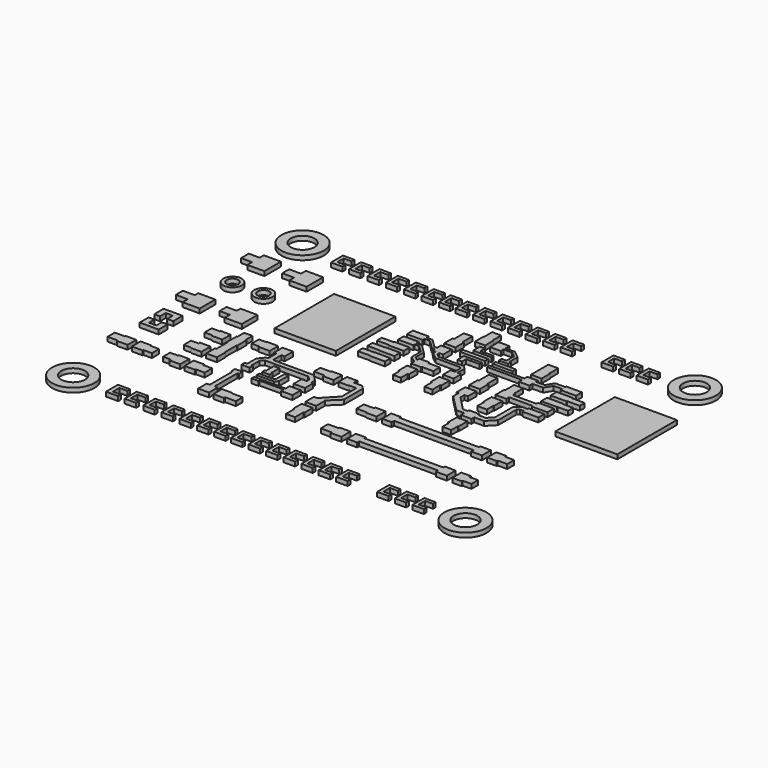
from build123d import *

# Parameters (mm, degrees)
F0_W     = 8.8383136317
F0_H     = 10.7280849479
F2_DEPTH = 0.635
F0_W_2   = 8.9478660375
F0_H_2   = 10.732548777
F0_W_3   = 3.4179408103
F0_H_3   = 0.6752701011
F0_W_4   = 1.5755221248
F0_H_4   = 1.3810726814
F0_W_5   = 1.7077755183
F0_H_5   = 1.243758481
F0_W_6   = 1.7230845988
F0_H_6   = 1.2770355679
F0_R     = 0.3036526341
F0_W_7   = 1.472780481
F0_H_7   = 1.2533185072
F0_R_2   = 0.3044951646
F0_W_8   = 1.8562953919
F0_H_8   = 0.8942730201
F0_W_9   = 1.5506837517
F0_H_9   = 0.9251098963
F0_W_10  = 1.4100596309
F0_H_10  = 0.5669312086
F0_W_11  = 1.561771147
F0_H_11  = 1.2164656073
F0_W_12  = 1.305432932
F0_H_12  = 1.5174094588
F0_W_13  = 1.1086538434
F0_H_13  = 1.3054329902
F0_W_14  = 1.5646023676
F0_H_14  = 1.2951530516
F0_W_15  = 1.2573283166
F0_H_15  = 1.1950880289
F0_W_16  = 1.378653571
F0_H_16  = 1.2574242428
F0_W_17  = 1.2773927301
F0_H_17  = 1.2361174449
F0_W_18  = 1.151248347
F0_H_18  = 1.3980204239
F0_W_19  = 3.6632483825
F0_H_19  = 0.4471028224
F0_W_20  = 1.1279918253
F0_H_20  = 1.2643169612
F0_W_21  = 1.2620901689
F0_H_21  = 2.1310206503
F0_W_22  = 1.202643849
F0_H_22  = 1.2692697346
F0_W_23  = 1.1741518974
F0_H_23  = 1.2878933921
F0_W_24  = 1.2717936188
F0_H_24  = 1.3373773545
F0_W_25  = 1.4900562819
F0_H_25  = 1.1629359797
F0_W_26  = 1.1306900997
F0_H_26  = 1.1970004998
F0_W_27  = 1.3690730557
F0_H_27  = 1.217473764
F0_W_28  = 1.0838713497
F0_H_28  = 1.3157110661
F0_W_29  = 1.3664499857
F0_H_29  = 0.4357985454
F0_W_30  = 1.2792297639
F0_H_30  = 0.5960047711
F1_R     = 3.0492368832
F1_R_2   = 1.7145
F3_DEPTH = 0.635
F1_R_3   = 1.3313448852
F1_R_4   = 0.8262831424
F1_R_5   = 1.3281430865
F1_R_6   = 0.8239920233
F1_R_7   = 3.048384159
F1_R_8   = 3.0501055082
F1_R_9   = 3.0482052647
F1_R_10  = 1.7111635464


# Not quite as in the source:
# - ends of sketch curves that miss each other by under 0.0002 mm in the source are joined
# - a feature names something its author has since deleted; it is built from what else it names


with BuildPart() as f2:
    # F0 (on Top) → F2 (new body)
    with BuildSketch(Plane.XY):
        with Locations((-10.1480917074, -1.0168242734)):
            Rectangle(F0_W, F0_H)
    extrude(amount=F2_DEPTH)


with BuildPart() as f2b:
    # F0 (on Top) → F2, piece 2 (new body)
    with BuildSketch(Plane.XY):
        with Locations((30.3083872423, -0.916500343)):
            Rectangle(F0_W_2, F0_H_2)
    extrude(amount=F2_DEPTH)


with BuildPart() as f2c:
    # F0 (on Top) → F2, piece 3 (new body)
    with BuildSketch(Plane.XY):
        with Locations((18.2702904567, -2.6805658126)):
            Rectangle(F0_W_3, F0_H_3)
        Polygon((15.1307059766, -0.3272882414), (15.1360724121, -1.9821051974), (16.4415054023, -1.9821051974), (16.4415054023, -0.3272882414), align=None)
        Polygon((19.9792608619, -2.3429307621), (19.9792608619, -3.0182008632), (19.9792608619, -3.1918291934), (22.220082581, -3.1918291934), (22.220082581, -2.0200230647), (19.9792608619, -2.0200230647), align=None)
        Polygon((15.1360724121, -1.9821051974), (15.0048257783, -1.9821051974), (15.0048257783, -3.5278119612), (16.5613200516, -3.5278119612), (16.5613200516, -3.0182008632), (16.5613200516, -2.3429307621), (16.5613200516, -1.9821051974), (16.4415054023, -1.9821051974), align=None)
    extrude(amount=F2_DEPTH)


with BuildPart() as f2d:
    # F0 (on Top) → F2, piece 4 (new body)
    with BuildSketch(Plane.XY):
        Polygon((-24.1649243981, 6.7577632144), (-26.6341436654, 6.7577632144), (-26.6341436654, 6.0122814029), (-26.6341436654, 4.6312087215), (-26.6341436654, 3.7751416676), (-24.1649243981, 3.7751416676), align=None)
        with Locations((-27.4219047278, 5.3217450622)):
            Rectangle(F0_W_4, F0_H_4)
    extrude(amount=F2_DEPTH)


with BuildPart() as f2e:
    # F0 (on Top) → F2, piece 5 (new body)
    with BuildSketch(Plane.XY):
        Polygon((-18.0774424225, 6.7577632144), (-20.5711107701, 6.7577632144), (-20.5711107701, 5.8749672025), (-20.5711107701, 4.6312087215), (-20.5711107701, 3.7751416676), (-18.0774424225, 3.7751416676), align=None)
        with Locations((-21.4249985293, 5.253087962)):
            Rectangle(F0_W_5, F0_H_5)
    extrude(amount=F2_DEPTH)


with BuildPart() as f2f:
    # F0 (on Top) → F2, piece 6 (new body)
    with BuildSketch(Plane.XY):
        Polygon((-24.1649243981, -5.0749327056), (-26.6341455281, -5.0749327056), (-26.6341455281, -5.6854607537), (-26.6341455281, -6.9624963216), (-26.6341455281, -7.8864200041), (-24.1649243981, -7.8864200041), align=None)
        with Locations((-27.4956878275, -6.3239785377)):
            Rectangle(F0_W_6, F0_H_6)
        with Locations((-27.8962515295, -6.3951537013)):
            Circle(F0_R, mode=Mode.SUBTRACT)
        with Locations((-27.8962515295, -6.3951537013)):
            Circle(F0_R)
    extrude(amount=F2_DEPTH)


with BuildPart() as f2g:
    # F0 (on Top) → F2, piece 7 (new body)
    with BuildSketch(Plane.XY):
        Polygon((-18.1018915027, -5.0504850224), (-20.5711107701, -5.0504850224), (-20.5711107701, -5.7091778144), (-20.5711107701, -6.9624963216), (-20.5711107701, -7.8864200041), (-18.1018915027, -7.8864200041), align=None)
        with Locations((-21.3075010106, -6.335837068)):
            Rectangle(F0_W_7, F0_H_7)
        with Locations((-21.5573497117, -6.3951537013)):
            Circle(F0_R_2, mode=Mode.SUBTRACT)
        with Locations((-21.5573497117, -6.3951537013)):
            Circle(F0_R_2)
    extrude(amount=F2_DEPTH)


with BuildPart() as f2h:
    # F0 (on Top) → F2, piece 8 (new body)
    with BuildSketch(Plane.XY):
        Polygon((19.9587028474, -3.7468951195), (19.9587028474, -3.9533996023), (19.9587028474, -4.5840349048), (19.9587028474, -4.8159109429), (22.220082581, -4.8159109429), (22.220082581, -3.7468951195), align=None)
        Polygon((15.0194698945, -9.1961659491), (15.0194698945, -8.5539119318), (14.3346317847, -8.5539119318), (12.3020727187, -6.4541599101), (12.3020727187, -5.7373908348), (11.4847198129, -5.7373908348), (11.4847198129, -6.742843182), (13.8865737244, -9.1961659491), align=None)
        Polygon((17.6625381124, -8.5858944803), (16.5613200516, -8.5858944803), (16.5613200516, -9.3020955101), (17.9853862302, -9.3020955101), (19.0944410861, -8.1543523612), (19.0944410861, -4.8597618444), (19.3846803159, -4.5840349048), (19.9587028474, -4.5840349048), (19.9587028474, -3.9533996023), (19.1347077489, -3.9533996023), (18.3828920126, -4.6720469973), (18.3828920126, -7.8655403551), align=None)
        Polygon((11.4847198129, -5.7373908348), (12.3020727187, -5.7373908348), (12.7952471375, -5.7373908348), (12.7952471375, -4.1965004057), (11.1816739663, -4.1965004057), (11.1816739663, -5.7373908348), align=None)
        Polygon((16.5613200516, -8.3131287247), (15.0194698945, -8.3131287247), (15.0194698945, -8.5539119318), (15.0194698945, -9.1961659491), (15.0194698945, -9.7933048382), (16.5613200516, -9.7933048382), (16.5613200516, -9.3020955101), (16.5613200516, -8.5858944803), align=None)
    extrude(amount=F2_DEPTH)


with BuildPart() as f2i:
    # F0 (on Top) → F2, piece 9 (new body)
    with BuildSketch(Plane.XY):
        Polygon((0.2071742638, 1.1828735005), (-1.987867523, 1.1828735005), (-1.987867523, 0.1507677225), (0.2071742638, 0.1507677225), (0.2071742638, 0.3949551319), (0.8484240971, 0.3949551319), (1.8542347467, -0.5398768699), (1.8542347467, -2.200213147), (2.7769438457, -2.8982465155), (2.7769438457, -3.4828390926), (4.2571197264, -3.4828390926), (4.2571197264, -3.3824450802), (5.9211971238, -3.3824450802), (5.9211971238, -2.2117714398), (4.2571197264, -2.2117714398), (4.2571197264, -1.9821051974), (2.7769438457, -1.9821051974), (2.7769438457, -2.3882756941), (2.2400394082, -1.9821051974), (2.2400394082, -0.4953329917), (0.995364855, 0.7406980731), (0.2071742638, 0.7406980731), align=None)
    extrude(amount=F2_DEPTH)


with BuildPart() as f2j:
    # F0 (on Top) → F2, piece 10 (new body)
    with BuildSketch(Plane.XY):
        with Locations((23.1571951881, 0.7704721793)):
            Rectangle(F0_W_8, F0_H_8)
        Polygon((22.2290474921, 1.3358424185), (19.9309624732, 1.3358424185), (19.9309624732, 0.2356950572), (22.2290474921, 0.2356950572), (22.2290474921, 0.3233356692), (22.2290474921, 1.2176086893), align=None)
    extrude(amount=F2_DEPTH)


with BuildPart() as f2k:
    # F0 (on Top) → F2, piece 11 (new body)
    with BuildSketch(Plane.XY):
        Polygon((0.2217109577, 2.9127409216), (-2.0460144151, 2.9127409216), (-2.0460144151, 1.8079516012), (0.2217109577, 1.8079516012), (0.2217109577, 2.1451261241), (0.2217109577, 2.5225197896), align=None)
        Polygon((3.6875456572, 0.4741872835), (3.1932978891, 0.4741872835), (3.1932978891, 0), (4.1236467659, -0.7333545946), (7.6851383783, -0.7333545946), (7.9177254811, -1.0095519247), (7.9177254811, -1.9821051974), (8.310216479, -1.9821051974), (8.310216479, -0.7042811485), (7.8159682453, -0.2681801561), (4.1963304393, -0.2681801561), (3.6875456572, 0.1533842151), align=None)
        Polygon((8.310216479, -1.9821051974), (7.9177254811, -1.9821051974), (7.3003736325, -1.9821051974), (7.3003736325, -3.3824450802), (8.8267270476, -3.3824450802), (8.8267270476, -1.9821051974), align=None)
        Polygon((2.6861303486, 2.047317801), (2.6861303486, 1.3202173682), (2.6861303486, 0.9452876402), (2.6861303486, 0.4741872835), (3.1932978891, 0.4741872835), (3.6875456572, 0.4741872835), (4.2571197264, 0.4741872835), (4.2571197264, 2.047317801), align=None)
        Polygon((1.0968204588, 2.5225197896), (0.2217109577, 2.5225197896), (0.2217109577, 2.1451261241), (1.0318105284, 2.1451261241), (2.2400394082, 0.9452876402), (2.6861303486, 0.9452876402), (2.6861303486, 1.3202173682), (2.3075305063, 1.3202173682), align=None)
    extrude(amount=F2_DEPTH)


with BuildPart() as f2l:
    # F0 (on Top) → F2, piece 12 (new body)
    with BuildSketch(Plane.XY):
        Polygon((11.3475334477, -0.1729048687), (11.3534005359, -1.9821051974), (12.6030265707, -1.9821051974), (12.5971594825, -0.1729048687), align=None)
        Polygon((11.3534005359, -1.9821051974), (11.1962100491, -1.9821051974), (11.1962100491, -3.5278121941), (12.7516370267, -3.5278121941), (12.7516370267, -1.9821051974), (12.6030265707, -1.9821051974), align=None)
    extrude(amount=F2_DEPTH)


with BuildPart() as f2m:
    # F0 (on Top) → F2, piece 13 (new body)
    with BuildSketch(Plane.XY):
        Polygon((0.1926377008, -3.9195087738), (-1.9442574121, -3.9195087738), (-1.9442574121, -3.9598466904), (-1.9442574121, -4.8703011125), (-1.9442574121, -4.9370778725), (0.1926377008, -4.9370778725), align=None)
        Polygon((-1.9442574121, -4.8703011125), (-1.9442574121, -3.9598466904), (-3.7691615199, -3.9657647046), (-3.766209022, -4.876209552), align=None)
    extrude(amount=F2_DEPTH)


with BuildPart() as f2n:
    # F0 (on Top) → F2, piece 14 (new body)
    with BuildSketch(Plane.XY):
        with Locations((23.0427468196, -1.0026553937)):
            Rectangle(F0_W_9, F0_H_9)
        Polygon((22.2674049437, -0.4488411068), (19.979858771, -0.4488411068), (19.979858771, -1.505690976), (22.2674049437, -1.505690976), (22.2674049437, -1.4652103418), (22.2674049437, -0.5401004455), align=None)
    extrude(amount=F2_DEPTH)


with BuildPart() as f2o:
    # F0 (on Top) → F2, piece 15 (new body)
    with BuildSketch(Plane.XY):
        Polygon((12.9254506901, 2.7643614449), (11.4117721096, 2.7643614449), (11.4117721096, 2.1974302363), (12.9254506901, 2.182893455), align=None)
        with Locations((10.7067422941, 2.4808958406)):
            Rectangle(F0_W_10, F0_H_10)
    extrude(amount=F2_DEPTH)


with BuildPart() as f2p:
    # F0 (on Top) → F2, piece 16 (new body)
    with BuildSketch(Plane.XY):
        with Locations((-7.6441639103, -22.3886007443)):
            Rectangle(F0_W_11, F0_H_11)
        Polygon((-8.4250494838, -21.6613095254), (-9.9290311337, -21.6613095254), (-9.9290311337, -23.2171528041), (-8.4250494838, -23.2171528041), (-8.4250494838, -23.0741333216), (-8.4250494838, -22.9968335479), (-8.4250494838, -21.7803679407), align=None)
    extrude(amount=F2_DEPTH)


with BuildPart() as f2q:
    # F0 (on Top) → F2, piece 17 (new body)
    with BuildSketch(Plane.XY):
        Polygon((16.4796393365, 4.3633985333), (15.0459473953, 4.3633985333), (15.0459473953, 2.822508337), (16.5723003447, 2.822508337), (16.5723003447, 4.3633985333), align=None)
        Polygon((15.0447645318, 5.9468320436), (15.0459473953, 4.3633985333), (16.4796393365, 4.3633985333), (16.4744893559, 5.9514685238), align=None)
    extrude(amount=F2_DEPTH)


with BuildPart() as f2r:
    # F0 (on Top) → F2, piece 18 (new body)
    with BuildSketch(Plane.XY):
        Polygon((10.0446669385, -14.3940951675), (8.6707342416, -14.3940951675), (8.6707342416, -16.0390567034), (10.0446669385, -16.0390567034), (10.0446669385, -15.5971283093), (10.0446669385, -14.6453212947), align=None)
        Polygon((21.4936956763, -14.3940951675), (21.4936956763, -14.6453212947), (21.4936956763, -15.2165759355), (21.4936956763, -15.5971283093), (21.4936956763, -16.0134024918), (23.0397265404, -16.0134024918), (23.0397265404, -14.3940951675), align=None)
        Polygon((21.4936956763, -14.6453212947), (10.0446669385, -14.6453212947), (10.0446669385, -15.5971283093), (21.4936956763, -15.5971283093), (21.4936956763, -15.2165759355), align=None)
    extrude(amount=F2_DEPTH)


with BuildPart() as f2s:
    # F0 (on Top) → F2, piece 19 (new body)
    with BuildSketch(Plane.XY):
        with Locations((0.126557512, -21.1234791204)):
            Rectangle(F0_W_12, F0_H_12)
        Polygon((0.9100104799, -18.8607927412), (-0.68040716, -18.8607927412), (-0.68040716, -20.3647743911), (-0.526158954, -20.3647743911), (0.779273978, -20.3647743911), (0.9100104799, -20.3647743911), align=None)
    extrude(amount=F2_DEPTH)


with BuildPart() as f2t:
    # F0 (on Top) → F2, piece 20 (new body)
    with BuildSketch(Plane.XY):
        Polygon((-11.5547031164, -9.5032630488), (-13.1438048556, -9.5032630488), (-13.1438048556, -9.6061397344), (-13.1438048556, -10.9115727246), (-13.1438048556, -11.0434694216), (-11.5547031164, -11.0434694216), align=None)
        with Locations((-13.6981317773, -10.2588562295)):
            Rectangle(F0_W_13, F0_H_13)
    extrude(amount=F2_DEPTH)


with BuildPart() as f2u:
    # F0 (on Top) → F2, piece 21 (new body)
    with BuildSketch(Plane.XY):
        with Locations((5.5193048902, -21.5424355119)):
            Rectangle(F0_W_14, F0_H_14)
        Polygon((7.8401621431, -20.7199398428), (6.301606074, -20.7199398428), (6.301606074, -20.8948589861), (6.301606074, -22.1900120378), (6.301606074, -22.3622191697), (7.8401621431, -22.3622191697), align=None)
    extrude(amount=F2_DEPTH)


with BuildPart() as f2v:
    # F0 (on Top) → F2, piece 22 (new body)
    with BuildSketch(Plane.XY):
        Polygon((6.3523445278, -15.9097872674), (6.3523445278, -14.6111982487), (4.868267102, -14.61601099), (4.8724627122, -15.9097872674), align=None)
        Polygon((7.8496243805, -14.3940951675), (6.3523445278, -14.3940951675), (6.3523445278, -14.6111982487), (6.3523445278, -15.9097872674), (6.3523445278, -16.0245187581), (7.8496243805, -16.0245187581), align=None)
    extrude(amount=F2_DEPTH)


with BuildPart() as f2w:
    # F0 (on Top) → F2, piece 23 (new body)
    with BuildSketch(Plane.XY):
        Polygon((-9.3910805881, -9.5154866576), (-10.919063352, -9.5154866576), (-10.919063352, -11.0312458128), (-10.5648478493, -11.0312458128), (-9.8827956244, -11.0312458128), (-9.3910805881, -11.0312458128), align=None)
        Polygon((-2.7940333821, -14.1650000587), (-3.0543725006, -14.1650000587), (-3.6163532641, -14.1650000587), (-3.6972675007, -14.1650000587), (-4.4386731461, -14.1650000587), (-4.4386731461, -15.6246172264), (-2.7940333821, -15.6246172264), align=None)
        Polygon((-10.9477292627, -15.0406714529), (-11.5720657632, -15.0406714529), (-11.9378063828, -15.0406714529), (-11.9378063828, -15.651864931), (-10.7491258532, -15.651864931), (-10.7491258532, -15.0406714529), align=None)
        Polygon((-9.8827956244, -11.0312458128), (-10.5648478493, -11.0312458128), (-10.5648478493, -12.5546036288), (-10.8463246506, -12.5546036288), (-11.5720657632, -13.4241807827), (-11.5720657632, -15.0406714529), (-10.9477292627, -15.0406714529), (-10.9477292627, -13.633874001), (-10.5298156054, -13.1804710254), (-4.2910656545, -13.1804710254), (-3.6972675007, -13.7277906761), (-3.6972675007, -14.1650000587), (-3.6163532641, -14.1650000587), (-3.0543725006, -14.1650000587), (-3.0543725006, -13.497619078), (-4.0043183329, -12.5286737457), (-9.8827956244, -12.5286737457), align=None)
    extrude(amount=F2_DEPTH)


with BuildPart() as f2x:
    # F0 (on Top) → F2, piece 24 (new body)
    with BuildSketch(Plane.XY):
        with Locations((25.8307503536, -21.5924680233)):
            Rectangle(F0_W_15, F0_H_15)
        Polygon((25.2020861953, -20.7239929587), (23.8380134106, -20.7239929587), (23.8380134106, -22.3497673869), (25.2020861953, -22.3497673869), (25.2020861953, -22.1900120378), (25.2020861953, -20.9949240088), align=None)
    extrude(amount=F2_DEPTH)


with BuildPart() as f2y:
    # F0 (on Top) → F2, piece 25 (new body)
    with BuildSketch(Plane.XY):
        with Locations((25.8914129809, -15.2540220879)):
            Rectangle(F0_W_16, F0_H_16)
        Polygon((25.2020861953, -14.3940951675), (23.8199867308, -14.3940951675), (23.8199867308, -16.0479769111), (25.2020861953, -16.0479769111), (25.2020861953, -15.8827342093), (25.2020861953, -14.6253099665), align=None)
    extrude(amount=F2_DEPTH)


with BuildPart() as f2z:
    # F0 (on Top) → F2, piece 26 (new body)
    with BuildSketch(Plane.XY):
        with Locations((15.830704011, -12.7195757814)):
            Rectangle(F0_W_17, F0_H_17)
        Polygon((16.5613200516, -10.5333924294), (15.0194698945, -10.5333924294), (15.0194698945, -12.1015170589), (15.192007646, -12.1015170589), (16.4694003761, -12.1015170589), (16.5613200516, -12.1015170589), align=None)
    extrude(amount=F2_DEPTH)


with BuildPart() as f2ba:
    # F0 (on Top) → F2, piece 27 (new body)
    with BuildSketch(Plane.XY):
        with Locations((8.0806224141, -6.2619601376)):
            Rectangle(F0_W_18, F0_H_18)
        Polygon((8.7976539508, -4.0365965106), (7.3294471949, -4.0365965106), (7.3294471949, -5.5629499257), (7.5049982406, -5.5629499257), (8.6562465876, -5.5629499257), (8.7976539508, -5.5629499257), align=None)
    extrude(amount=F2_DEPTH)


with BuildPart() as f2bb:
    # F0 (on Top) → F2, piece 28 (new body)
    with BuildSketch(Plane.XY):
        with Locations((13.214323204, 1.4105285518)):
            Rectangle(F0_W_19, F0_H_19)
        Polygon((15.0459473953, 2.1538201254), (15.0459473953, 1.634079963), (15.0459473953, 1.1869771406), (15.0459473953, 0.6274664775), (16.5723003447, 0.6274664775), (16.5723003447, 1.1869771406), (16.5723003447, 1.8014175585), (16.5723003447, 2.1538201254), align=None)
        Polygon((17.8238973022, 1.7969222972), (16.5723003447, 1.8014175585), (16.5723003447, 1.1869771406), (18.0788311207, 1.1869771406), (18.7606476247, 2.2811817471), (19.979858771, 2.2908467832), (19.979858771, 2.8829667717), (18.4969167827, 2.8829667717), align=None)
        Polygon((11.3826990128, 1.6429694369), (10.0017124787, 1.6429694369), (10.0017124787, 1.1869771406), (11.3826990128, 1.1869771406), (11.3826990128, 1.634079963), align=None)
    extrude(amount=F2_DEPTH)


with BuildPart() as f2bc:
    # F0 (on Top) → F2, piece 29 (new body)
    with BuildSketch(Plane.XY):
        Polygon((-4.4309725054, -16.344146803), (-4.4309725054, -17.083434388), (-4.4309725054, -17.4136292189), (-4.4309725054, -17.8654398769), (-2.8145913966, -17.8654398769), (-2.8145913966, -16.344146803), align=None)
        Polygon((-4.4309725054, -17.083434388), (-7.9242177308, -17.0860216022), (-7.9242177308, -17.4136292189), (-4.4309725054, -17.4136292189), align=None)
        Polygon((-7.9242177308, -17.0860216022), (-8.9754704386, -17.0860216022), (-8.9754704386, -17.5587870181), (-7.9242177308, -17.5587870181), (-7.9242177308, -17.4136292189), align=None)
    extrude(amount=F2_DEPTH)


with BuildPart() as f2bd:
    # F0 (on Top) → F2, piece 30 (new body)
    with BuildSketch(Plane.XY):
        Polygon((2.844377108, 5.9831562107), (2.8500770476, 4.225498531), (4.0582967922, 4.225498531), (4.0582967922, 5.9870928526), align=None)
        Polygon((2.8500770476, 4.225498531), (2.6342689525, 4.225498531), (2.6342689525, 2.686942229), (4.2571197264, 2.686942229), (4.2571197264, 4.225498531), (4.0582967922, 4.225498531), align=None)
    extrude(amount=F2_DEPTH)


with BuildPart() as f2be:
    # F0 (on Top) → F2, piece 31 (new body)
    with BuildSketch(Plane.XY):
        Polygon((-17.3945631832, -18.2323865592), (-18.9225450158, -18.2323865592), (-18.9225450158, -18.3797925711), (-18.9225450158, -19.6441095322), (-18.9225450158, -19.8842734098), (-17.3945631832, -19.8842734098), align=None)
        with Locations((-19.4865409285, -19.0119510517)):
            Rectangle(F0_W_20, F0_H_20)
    extrude(amount=F2_DEPTH)


with BuildPart() as f2bf:
    # F0 (on Top) → F2, piece 32 (new body)
    with BuildSketch(Plane.XY):
        Polygon((-24.9740947038, -18.3143094182), (-26.5295226127, -18.3143094182), (-26.5295226127, -18.4495858848), (-26.5295226127, -19.7447389364), (-26.5295226127, -19.8842734098), (-24.9740947038, -19.8842734098), align=None)
        Polygon((-26.5295226127, -19.7447389364), (-26.5295226127, -18.4495858848), (-27.963930741, -18.4495858848), (-27.963930741, -19.7319835424), align=None)
    extrude(amount=F2_DEPTH)


with BuildPart() as f2bg:
    # F0 (on Top) → F2, piece 33 (new body)
    with BuildSketch(Plane.XY):
        Polygon((-16.5618881583, -14.3940951675), (-16.7589224875, -14.3940951675), (-16.7589224875, -15.970973298), (-15.2187170461, -15.970973298), (-15.2187170461, -14.3940951675), (-15.2997979894, -14.3940951675), align=None)
        with Locations((-15.9308430739, -13.3285848424)):
            Rectangle(F0_W_21, F0_H_21)
        with Locations((-15.9536334686, -10.0249154493)):
            Rectangle(F0_W_22, F0_H_22)
        Polygon((-16.6226383299, -12.2630745173), (-16.5618881583, -12.2630745173), (-15.2997979894, -12.2630745173), (-15.2187170461, -12.2630745173), (-15.2187170461, -10.6595503166), (-15.3523115441, -10.6595503166), (-16.5549553931, -10.6595503166), (-16.6611876339, -10.6595503166), (-16.6611876339, -12.2630745173), align=None)
    extrude(amount=F2_DEPTH)


with BuildPart() as f2bh:
    # F0 (on Top) → F2, piece 34 (new body)
    with BuildSketch(Plane.XY):
        Polygon((19.979858771, 3.0471829232), (19.979858771, 2.8829667717), (19.9802108109, 2.2908495739), (19.979858771, 2.2908467832), (19.979858771, 1.9714832306), (22.2290474921, 1.9714832306), (22.2290474921, 3.0471829232), align=None)
    extrude(amount=F2_DEPTH)


with BuildPart() as f2bi:
    # F0 (on Top) → F2, piece 35 (new body)
    with BuildSketch(Plane.XY):
        Polygon((0.2071742056, -2.204178134), (-1.9587941933, -2.204178134), (-1.9587941933, -2.2656874257), (-1.9587941933, -3.1918291934), (-1.9587941933, -3.2508205622), (0.2071742056, -3.2508205622), align=None)
        Polygon((-1.9587941933, -3.1918291934), (-1.9587941933, -2.2656874257), (-3.7309079399, -2.2714342451), (-3.7279045697, -3.1975662731), align=None)
    extrude(amount=F2_DEPTH)


with BuildPart() as f2bj:
    # F0 (on Top) → F2, piece 36 (new body)
    with BuildSketch(Plane.XY):
        Polygon((-11.3292904571, -21.6958839446), (-11.6712236777, -21.6958839446), (-12.1072120965, -21.6958839446), (-12.1072120965, -23.2344400138), (-10.5513688177, -23.2344400138), (-10.5513688177, -21.6958839446), (-10.9892021865, -21.6958839446), align=None)
        Polygon((-10.747930035, -16.9231463224), (-11.848077178, -16.9231463224), (-11.848077178, -17.5465643406), (-11.6712236777, -17.5465643406), (-11.3292904571, -17.5465643406), (-10.9892021865, -17.5465643406), (-10.747930035, -17.5465643406), align=None)
        Polygon((-11.3292904571, -17.5465643406), (-11.6712236777, -17.5465643406), (-11.6712236777, -21.6958839446), (-11.3292904571, -21.6958839446), (-10.9892021865, -21.6958839446), (-10.9892021865, -17.5465643406), align=None)
    extrude(amount=F2_DEPTH)


with BuildPart() as f2bk:
    # F0 (on Top) → F2, piece 37 (new body)
    with BuildSketch(Plane.XY):
        with Locations((-19.5096209645, -11.4571540616)):
            Rectangle(F0_W_23, F0_H_23)
        Polygon((-17.4526702613, -10.6903873384), (-18.9225450158, -10.6903873384), (-18.9225450158, -10.8132073656), (-18.9225450158, -12.1011007577), (-18.9225450158, -12.2219584882), (-17.4526702613, -12.2219584882), align=None)
    extrude(amount=F2_DEPTH)


with BuildPart() as f2bl:
    # F0 (on Top) → F2, piece 38 (new body)
    with BuildSketch(Plane.XY):
        with Locations((-14.5950429142, -19.0813457593)):
            Rectangle(F0_W_24, F0_H_24)
        Polygon((-15.2309397236, -18.2201620191), (-16.7589224875, -18.2201620191), (-16.7589224875, -19.8842734098), (-15.2309397236, -19.8842734098), (-15.2309397236, -19.7500344366), (-15.2309397236, -18.4126570821), align=None)
    extrude(amount=F2_DEPTH)


with BuildPart() as f2bm:
    # F0 (on Top) → F2, piece 39 (new body)
    with BuildSketch(Plane.XY):
        Polygon((-1.4929026365, -10.5629600585), (-3.0314589385, -10.5629600585), (-3.0314589385, -10.6892511249), (-3.0314589385, -11.8521871045), (-3.0314589385, -12.0842298493), (-1.4929026365, -12.0842298493), align=None)
        with Locations((-3.7764870794, -11.2707191147)):
            Rectangle(F0_W_25, F0_H_25)
    extrude(amount=F2_DEPTH)


with BuildPart() as f2bn:
    # F0 (on Top) → F2, piece 40 (new body)
    with BuildSketch(Plane.XY):
        Polygon((4.2571197264, -4.1674268432), (2.7794595808, -4.1674268432), (2.7794595808, -5.7228538208), (2.9411225114, -5.7228538208), (4.0718126111, -5.7228538208), (4.2571197264, -5.7228538208), align=None)
        with Locations((3.5064675612, -6.3213540707)):
            Rectangle(F0_W_26, F0_H_26)
    extrude(amount=F2_DEPTH)


with BuildPart() as f2bo:
    # F0 (on Top) → F2, piece 41 (new body)
    with BuildSketch(Plane.XY):
        Polygon((0.7025651284, -12.1015170589), (0.7025651284, -12.0323011652), (0.7025651284, -11.1660528928), (0.7025651284, -10.5629600585), (-0.7841295446, -10.5629600585), (-0.7841295446, -12.1015170589), align=None)
        Polygon((-0.1911776483, -16.6826117784), (-0.6631200667, -16.6826117784), (-0.6631200667, -18.2323865592), (0.9100104799, -18.2323865592), (0.9100104799, -16.6826117784), (0.7765043993, -16.6826117784), align=None)
        Polygon((1.7395425821, -14.6358472122), (-0.1911776483, -16.6826117784), (0.7765043993, -16.6826117784), (2.3942143215, -15.1143586263), (2.3942143215, -11.6536887256), (1.877269542, -11.1660528928), (0.7025651284, -11.1660528928), (0.7025651284, -12.0323011652), (1.7395425821, -12.0323011652), align=None)
    extrude(amount=F2_DEPTH)


with BuildPart() as f2bp:
    # F0 (on Top) → F2, piece 42 (new body)
    with BuildSketch(Plane.XY):
        Polygon((5.1523471608, 8.1878244079), (5.1571799638, 6.6975606605), (6.4526102506, 6.6975606605), (6.4477638243, 8.1920253378), align=None)
        Polygon((5.1571799638, 6.6975606605), (5.0717568956, 6.6975606605), (5.0717568956, 5.1590045914), (6.5584513359, 5.1590045914), (6.5584513359, 6.6975606605), (6.4526102506, 6.6975606605), align=None)
    extrude(amount=F2_DEPTH)


with BuildPart() as f2bq:
    # F0 (on Top) → F2, piece 43 (new body)
    with BuildSketch(Plane.XY):
        Polygon((10.0874919444, -20.7545142621), (8.6526582018, -20.7545142621), (8.6526582018, -22.3276447505), (10.0874919444, -22.3276447505), (10.0874919444, -21.967113018), (10.0874919444, -21.5410795063), (10.0874919444, -21.0208911449), align=None)
        Polygon((21.473351866, -20.7414086908), (21.473351866, -21.0208911449), (21.473351866, -21.5410795063), (21.473351866, -21.967113018), (21.473351866, -22.3449338228), (23.0357609689, -22.3449338228), (23.0357609689, -20.7414086908), align=None)
        Polygon((21.473351866, -21.0208911449), (10.0874919444, -21.0208911449), (10.0874919444, -21.5410795063), (10.0874919444, -21.967113018), (21.473351866, -21.967113018), (21.473351866, -21.5410795063), align=None)
    extrude(amount=F2_DEPTH)


with BuildPart() as f2br:
    # F0 (on Top) → F2, piece 44 (new body)
    with BuildSketch(Plane.XY):
        Polygon((-22.8081271052, -18.3143094182), (-24.3635531515, -18.3143094182), (-24.3635531515, -19.8842734098), (-22.8081271052, -19.8842734098), (-22.8081271052, -19.7447389364), (-22.8081271052, -18.4495858848), align=None)
        Polygon((-21.574722603, -18.4495858848), (-22.8081271052, -18.4495858848), (-22.8081271052, -19.7447389364), (-21.574722603, -19.7465121746), align=None)
    extrude(amount=F2_DEPTH)


with BuildPart() as f2bs:
    # F0 (on Top) → F2, piece 45 (new body)
    with BuildSketch(Plane.XY):
        Polygon((-6.927463226, -16.1111559719), (-7.9364422709, -16.1111559719), (-7.9364422709, -16.5735892951), (-6.4967493765, -16.5735892951), (-6.1236107722, -16.1370877177), (-6.1236107722, -15.3591651469), (-6.1236107722, -14.4160203636), (-6.6946204752, -14.4160203636), (-6.7286612466, -15.3591651469), (-6.7286612466, -15.920996666), align=None)
        Polygon((-7.9364422709, -16.1110907793), (-9.0243658051, -16.1110907793), (-9.0243658051, -16.5743324906), (-7.9364422709, -16.5743324906), (-7.9364422709, -16.5735892951), align=None)
    extrude(amount=F2_DEPTH)


with BuildPart() as f2bt:
    # F0 (on Top) → F2, piece 46 (new body)
    with BuildSketch(Plane.XY):
        Polygon((0.2362475643, -0.5324574886), (-1.9587941933, -0.5324574886), (-1.9587941933, -0.6393476657), (-1.9587941933, -1.505690976), (-1.9587941933, -1.6081733629), (0.2362475643, -1.6081733629), align=None)
        Polygon((-1.9587941933, -1.505690976), (-1.9587941933, -0.6393476657), (-3.7064561922, -0.6450151901), (-3.7036467416, -1.5113493896), align=None)
    extrude(amount=F2_DEPTH)


with BuildPart() as f2bu:
    # F0 (on Top) → F2, piece 47 (new body)
    with BuildSketch(Plane.XY):
        with Locations((15.7849160023, -6.3170541544)):
            Rectangle(F0_W_27, F0_H_27)
        Polygon((16.5613200516, -4.2110369541), (14.9902896956, -4.2110369541), (14.9902896956, -5.7083172724), (15.1003794745, -5.7083172724), (16.4694525301, -5.7083172724), (16.5613200516, -5.7083172724), align=None)
    extrude(amount=F2_DEPTH)


with BuildPart() as f2bv:
    # F0 (on Top) → F2, piece 48 (new body)
    with BuildSketch(Plane.XY):
        Polygon((-17.4190104008, -14.3696470186), (-18.946994096, -14.3696470186), (-18.946994096, -14.6164000034), (-18.946994096, -15.9321110696), (-18.946994096, -16.0198677331), (-17.4190104008, -16.0198677331), align=None)
        with Locations((-19.4889297709, -15.2742555365)):
            Rectangle(F0_W_28, F0_H_28)
    extrude(amount=F2_DEPTH)


with BuildPart() as f2bw:
    # F0 (on Top) → F2, piece 49 (new body)
    with BuildSketch(Plane.XY):
        Polygon((10.13205276, 6.0441586718), (8.7976539508, 6.0441586718), (8.7976539508, 5.6995763443), (10.0389868021, 5.6995763443), (10.7623770699, 5.1293584511), (10.7623770699, 3.7751416676), (11.1962100491, 3.7751416676), (11.1962100491, 5.2053285763), align=None)
        Polygon((8.7976539508, 6.7494222894), (7.2499373928, 6.7494222894), (7.2499373928, 5.193578545), (8.7976539508, 5.193578545), (8.7976539508, 5.6995763443), (8.7976539508, 6.0441586718), align=None)
        Polygon((11.3972360268, 3.7751416676), (11.1962100491, 3.7751416676), (10.7623770699, 3.7751416676), (10.0446669385, 3.7751416676), (10.0446669385, 3.2837276813), (11.3972360268, 3.2837276813), align=None)
    extrude(amount=F2_DEPTH)


with BuildPart() as f2bx:
    # F0 (on Top) → F2, piece 50 (new body)
    with BuildSketch(Plane.XY):
        Polygon((7.5595467351, 1.2089344673), (7.5595467351, 1.6447330127), (6.3207859275, 1.6447330127), (6.301606074, 1.6306909965), (6.301606074, 0.4897392937), (6.9797504693, 0.4897392937), (6.9797504693, 1.2105697533), align=None)
        with Locations((8.242771728, 1.42683374)):
            Rectangle(F0_W_29, F0_H_29)
    extrude(amount=F2_DEPTH)


with BuildPart() as f2by:
    # F0 (on Top) → F2, piece 51 (new body)
    with BuildSketch(Plane.XY):
        Polygon((-8.86316659, -14.5700862631), (-8.8489583328, -15.0651196018), (-8.0597717315, -15.0651196018), (-8.0597717315, -13.6363320053), (-8.8659180328, -13.6363320053), (-8.8659180328, -14.5700862631), align=None)
        Polygon((-8.8489583328, -15.0651196018), (-9.0243648738, -15.0651196018), (-9.0243648738, -15.5785223469), (-7.9364422709, -15.5785223469), (-7.9364422709, -15.0651196018), (-8.0597717315, -15.0651196018), align=None)
    extrude(amount=F2_DEPTH)


with BuildPart() as f2bz:
    # F0 (on Top) → F2, piece 52 (new body)
    with BuildSketch(Plane.XY):
        Polygon((7.6467669569, 2.182893455), (7.6467669569, 2.7788982261), (5.3249350749, 2.7713687159), (5.3249350749, 2.182893455), align=None)
        with Locations((8.2863818388, 2.4808958406)):
            Rectangle(F0_W_30, F0_H_30)
    extrude(amount=F2_DEPTH)


with BuildPart() as f2ca:
    # F0 (on Top) → F2, piece 53 (new body)
    with BuildSketch(Plane.XY):
        Polygon((8.9114597067, 3.7751416676), (7.5740832835, 3.7751416676), (7.5740832835, 3.7286267596), (7.5740832835, 3.3370288078), (8.9114597067, 3.3370288078), align=None)
        Polygon((7.5740832835, 3.3370288078), (7.5740832835, 3.7286267596), (7.0229395034, 3.7286267596), (7.0202836274, 4.5476039974), (6.286450959, 4.5476039974), (6.2902960926, 3.3619021997), (6.3207859275, 3.3370288078), align=None)
    extrude(amount=F2_DEPTH)


with BuildPart() as f3:
    # F1 (on Top) → F3 (new body)
    with BuildSketch(Plane.XY):
        with Locations((-25.1280814409, 11.860800907)):
            Circle(F1_R)
        with Locations((-25.1280814409, 11.860800907)):
            Circle(F1_R_2, mode=Mode.SUBTRACT)
    extrude(amount=F3_DEPTH)


with BuildPart() as f3b:
    # F1 (on Top) → F3, piece 2 (new body)
    with BuildSketch(Plane.XY):
        Polygon((-17.9852191359, 10.119907558), (-17.9852191359, 10.6416475028), (-19.1280623784, 10.6416475028), (-19.1280623784, 11.7764876743), (-17.9852191359, 11.7764876743), (-17.9852191359, 12.2842919081), (-19.6397453547, 12.2842919081), (-19.6397453547, 10.119907558), align=None)
    extrude(amount=F3_DEPTH)


with BuildPart() as f3c:
    # F1 (on Top) → F3, piece 3 (new body)
    with BuildSketch(Plane.XY):
        Polygon((-15.3927598149, 10.1249180734), (-15.3927598149, 10.636985302), (-16.5286979902, 10.636985302), (-16.5286979902, 11.7811498751), (-15.3927598149, 11.7811498751), (-15.3927598149, 12.2842919081), (-17.0444883406, 12.2842919081), (-17.0444883406, 10.1249180734), align=None)
    extrude(amount=F3_DEPTH)


with BuildPart() as f3d:
    # F1 (on Top) → F3, piece 4 (new body)
    with BuildSketch(Plane.XY):
        Polygon((-12.7073843032, 10.1178530604), (-12.7073843032, 10.636985302), (-13.8558138488, 10.636985302), (-13.8558138488, 11.7811498751), (-12.7073843032, 11.7811498751), (-12.7073843032, 12.2806448489), (-14.3635068089, 12.2806448489), (-14.3635068089, 10.1178530604), align=None)
    extrude(amount=F3_DEPTH)


with BuildPart() as f3e:
    # F1 (on Top) → F3, piece 5 (new body)
    with BuildSketch(Plane.XY):
        Polygon((-10.0806783885, 10.1150907576), (-10.0806783885, 10.6336586177), (-11.2359238031, 10.6336586177), (-11.2359238031, 11.7844765593), (-10.0806783885, 11.7844765593), (-10.0806783885, 12.2832302004), (-11.7255970836, 12.2832302004), (-11.7255970836, 10.1150907576), align=None)
    extrude(amount=F3_DEPTH)


with BuildPart() as f3f:
    # F1 (on Top) → F3, piece 6 (new body)
    with BuildSketch(Plane.XY):
        Polygon((-7.4770804495, 10.1221762598), (-7.4770804495, 10.6387510896), (-8.613090981, 10.6387510896), (-8.613090981, 11.7793840875), (-7.4770804495, 11.7793840875), (-7.4770804495, 12.2761446983), (-9.1252494603, 12.2761446983), (-9.1252494603, 10.1221762598), align=None)
    extrude(amount=F3_DEPTH)


with BuildPart() as f3g:
    # F1 (on Top) → F3, piece 7 (new body)
    with BuildSketch(Plane.XY):
        Polygon((-4.9168951809, 10.1181417704), (-4.9168951809, 10.6387510896), (-6.0715493837, 10.6387510896), (-6.0715493837, 11.7793840875), (-4.9168951809, 11.7793840875), (-4.9168951809, 12.2836306691), (-6.555525586, 12.2836306691), (-6.555525586, 10.1181417704), align=None)
    extrude(amount=F3_DEPTH)


with BuildPart() as f3h:
    # F1 (on Top) → F3, piece 8 (new body)
    with BuildSketch(Plane.XY):
        Polygon((-2.4819634855, 10.1518444717), (-2.4819634855, 10.6337405741), (-3.6248330353, 10.6337405741), (-3.6248330353, 11.7843946029), (-2.4819634855, 11.7843946029), (-2.4819634855, 12.3004820198), (-4.1204001755, 12.3004820198), (-4.1204001755, 10.1518444717), align=None)
    extrude(amount=F3_DEPTH)


with BuildPart() as f3i:
    # F1 (on Top) → F3, piece 9 (new body)
    with BuildSketch(Plane.XY):
        Polygon((-0.0520404428, 10.134993121), (-0.0520404428, 10.643761605), (-1.2027740805, 10.643761605), (-1.2027740805, 11.774373572), (-0.0520404428, 11.774373572), (-0.0520404428, 12.2752040625), (-1.6937032342, 12.2752040625), (-1.6937032342, 10.134993121), align=None)
    extrude(amount=F3_DEPTH)


with BuildPart() as f3j:
    # F1 (on Top) → F3, piece 10 (new body)
    with BuildSketch(Plane.XY):
        Polygon((2.4647125974, 10.134993121), (2.4647125974, 10.6428209692), (1.3277569459, 10.6428209692), (1.3277569459, 11.7753142078), (2.4647125974, 11.7753142078), (2.4647125974, 12.2920572758), (0.8172541857, 12.2920572758), (0.8172541857, 10.134993121), align=None)
    extrude(amount=F3_DEPTH)


with BuildPart() as f3k:
    # F1 (on Top) → F3, piece 11 (new body)
    with BuildSketch(Plane.XY):
        Polygon((5.0148777664, 10.1302266121), (5.0148777664, 10.6371231377), (3.8762755366, 10.6371231377), (3.8762755366, 11.7810120393), (5.0148777664, 11.7810120393), (5.0148777664, 12.2920572758), (3.3676233143, 12.2920572758), (3.3676233143, 10.1302266121), align=None)
    extrude(amount=F3_DEPTH)


with BuildPart() as f3l:
    # F1 (on Top) → F3, piece 12 (new body)
    with BuildSketch(Plane.XY):
        Polygon((7.52496114, 10.1302266121), (7.52496114, 10.6371231377), (6.3929172838, 10.6371231377), (6.3929172838, 11.7810120393), (7.52496114, 11.7810120393), (7.52496114, 12.2920572758), (5.8728037402, 12.2920572758), (5.8728037402, 10.1302266121), align=None)
    extrude(amount=F3_DEPTH)


with BuildPart() as f3m:
    # F1 (on Top) → F3, piece 13 (new body)
    with BuildSketch(Plane.XY):
        Polygon((10.0689318497, 10.1302266121), (10.0689318497, 10.6371231377), (8.9200534066, 10.6371231377), (8.9200534066, 11.7810120393), (10.0689318497, 11.7810120393), (10.0689318497, 12.2920572758), (8.4174652584, 12.2920572758), (8.4174652584, 10.1302266121), align=None)
    extrude(amount=F3_DEPTH)


with BuildPart() as f3n:
    # F1 (on Top) → F3, piece 14 (new body)
    with BuildSketch(Plane.XY):
        Polygon((12.5951680529, 10.1302266121), (12.5951680529, 10.6430817395), (11.4476125245, 10.6430817395), (11.4476125245, 11.7750534375), (12.5951680529, 11.7750534375), (12.5951680529, 12.2920572758), (10.9493187629, 12.2920572758), (10.9493187629, 10.1302266121), align=None)
    extrude(amount=F3_DEPTH)


with BuildPart() as f3o:
    # F1 (on Top) → F3, piece 15 (new body)
    with BuildSketch(Plane.XY):
        Polygon((21.0338877514, 10.1302266121), (21.0338877514, 10.6438789517), (19.8909604596, 10.6438789517), (19.8909604596, 11.7742562254), (21.0338877514, 11.7742562254), (21.0338877514, 12.2920572758), (19.3763882853, 12.2920572758), (19.3763882853, 10.1302266121), align=None)
    extrude(amount=F3_DEPTH)


with BuildPart() as f3p:
    # F1 (on Top) → F3, piece 16 (new body)
    with BuildSketch(Plane.XY):
        Polygon((23.5660821199, 10.1302266121), (23.5660821199, 10.6438789517), (22.4200777383, 10.6438789517), (22.4200777383, 11.7742562254), (23.5660821199, 11.7742562254), (23.5660821199, 12.2920572758), (21.9215443358, 12.2920572758), (21.9215443358, 10.1302266121), align=None)
    extrude(amount=F3_DEPTH)


with BuildPart() as f3q:
    # F1 (on Top) → F3, piece 17 (new body)
    with BuildSketch(Plane.XY):
        Polygon((26.1028362438, 10.1128723472), (26.1028362438, 10.6357689947), (24.9714666651, 10.6357689947), (24.9714666651, 11.7823661823), (26.1028362438, 11.7823661823), (26.1028362438, 12.2822672129), (24.4554048404, 12.2822672129), (24.4554048404, 10.1128723472), align=None)
    extrude(amount=F3_DEPTH)


with BuildPart() as f3r:
    # F1 (on Top) → F3, piece 18 (new body)
    with BuildSketch(Plane.XY):
        with Locations((-20.8602063358, -0.5315141752)):
            Circle(F1_R_3)
        with Locations((-20.8602063358, -0.5315141752)):
            Circle(F1_R_4, mode=Mode.SUBTRACT)
    extrude(amount=F3_DEPTH)


with BuildPart() as f3s:
    # F1 (on Top) → F3, piece 19 (new body)
    with BuildSketch(Plane.XY):
        with Locations((-25.3215543926, -0.5315141752)):
            Circle(F1_R_5)
        with Locations((-25.3215543926, -0.5315141752)):
            Circle(F1_R_6, mode=Mode.SUBTRACT)
    extrude(amount=F3_DEPTH)


with BuildPart() as f3t:
    # F1 (on Top) → F3, piece 20 (new body)
    with BuildSketch(Plane.XY):
        Polygon((15.1273144875, 10.1302266121), (15.1273144875, 10.6438789517), (13.9833096554, 10.6438789517), (13.9833096554, 11.7742562254), (15.1273144875, 11.7742562254), (15.1273144875, 12.2920572758), (13.4744335664, 12.2920572758), (13.4744335664, 10.1302266121), align=None)
    extrude(amount=F3_DEPTH)


with BuildPart() as f3u:
    # F1 (on Top) → F3, piece 21 (new body)
    with BuildSketch(Plane.XY):
        Polygon((-27.3048579693, -12.1609065682), (-26.4577865601, -12.1609065682), (-26.4577865601, -11.1413566628), (-25.4396013916, -11.1413566628), (-25.4396013916, -12.1609065682), (-24.5648436248, -12.1609065682), (-24.5822425817, -10.4732096245), (-27.3048579693, -10.4723736446), align=None)
    extrude(amount=F3_DEPTH)


with BuildPart() as f3v:
    # F1 (on Top) → F3, piece 22 (new body)
    with BuildSketch(Plane.XY):
        Polygon((-27.3048579693, -13.1805157289), (-27.3048579693, -14.7774610668), (-24.5648436248, -14.7774610668), (-24.5648436248, -13.1718721241), (-25.4032723606, -13.1805157289), (-25.4032723606, -14.1572393477), (-26.4577865601, -14.1572393477), (-26.4577865601, -13.1805157289), align=None)
    extrude(amount=F3_DEPTH)


with BuildPart() as f3w:
    # F1 (on Top) → F3, piece 23 (new body)
    with BuildSketch(Plane.XY):
        with Locations((-25.1280814409, -29.5057427138)):
            Circle(F1_R_7)
        with Locations((-25.1280814409, -29.5057427138)):
            Circle(F1_R_2, mode=Mode.SUBTRACT)
    extrude(amount=F3_DEPTH)


with BuildPart() as f3x:
    # F1 (on Top) → F3, piece 24 (new body)
    with BuildSketch(Plane.XY):
        with Locations((31.4591582865, -29.5057427138)):
            Circle(F1_R_8)
        with Locations((31.4591582865, -29.5057427138)):
            Circle(F1_R_2, mode=Mode.SUBTRACT)
    extrude(amount=F3_DEPTH)


with BuildPart() as f3y:
    # F1 (on Top) → F3, piece 25 (new body)
    with BuildSketch(Plane.XY):
        with Locations((31.4591582865, 11.860800907)):
            Circle(F1_R_9)
        with Locations((31.4591582865, 11.860800907)):
            Circle(F1_R_10, mode=Mode.SUBTRACT)
    extrude(amount=F3_DEPTH)


with BuildPart() as f3z:
    # F1 (on Top) → F3, piece 26 (new body)
    with BuildSketch(Plane.XY):
        Polygon((-17.9797558281, -30.3225685107), (-17.9797558281, -29.8351127419), (-19.1335256862, -29.8351127419), (-19.1335256862, -28.6715685107), (-17.9797558281, -28.6715685107), (-17.9797558281, -28.1635685107), (-19.7457335889, -28.1635685107), (-19.7457335889, -30.3225685107), align=None)
    extrude(amount=F3_DEPTH)


with BuildPart() as f3ba:
    # F1 (on Top) → F3, piece 27 (new body)
    with BuildSketch(Plane.XY):
        Polygon((-15.383163218, -30.3377714008), (-15.383163218, -29.8303193233), (-16.538294587, -29.8303193233), (-16.538294587, -28.6763619293), (-15.383163218, -28.6763619293), (-15.383163218, -28.159590438), (-17.0402289025, -28.1640775053), (-17.0402289025, -30.3426037473), align=None)
    extrude(amount=F3_DEPTH)


with BuildPart() as f3bb:
    # F1 (on Top) → F3, piece 28 (new body)
    with BuildSketch(Plane.XY):
        Polygon((-12.7099376054, -30.3342249244), (-12.7099376054, -29.8187434673), (-13.8532605467, -29.8187434673), (-13.8532605467, -28.6879377852), (-12.7099376054, -28.6879377852), (-12.7099376054, -28.1847044826), (-14.3517944962, -28.1847044826), (-14.3517944962, -30.3342249244), align=None)
    extrude(amount=F3_DEPTH)


with BuildPart() as f3bc:
    # F1 (on Top) → F3, piece 29 (new body)
    with BuildSketch(Plane.XY):
        Polygon((-10.0942688802, -30.3349271417), (-10.0942688802, -29.8192289434), (-11.2223333114, -29.8192289434), (-11.2223333114, -28.6874523091), (-10.0942688802, -28.6874523091), (-10.0942688802, -28.1837783197), (-11.7476917803, -28.1837783197), (-11.7476917803, -30.3349271417), align=None)
    extrude(amount=F3_DEPTH)


with BuildPart() as f3bd:
    # F1 (on Top) → F3, piece 30 (new body)
    with BuildSketch(Plane.XY):
        Polygon((-7.482148017, -30.3272289434), (-7.482148017, -29.8192289434), (-8.6080234135, -29.8192289434), (-8.6080234135, -28.6874523091), (-7.482148017, -28.6874523091), (-7.482148017, -28.1837783197), (-9.144987911, -28.1837783197), (-9.144987911, -30.3272289434), align=None)
    extrude(amount=F3_DEPTH)


with BuildPart() as f3be:
    # F1 (on Top) → F3, piece 31 (new body)
    with BuildSketch(Plane.XY):
        Polygon((-4.9299663562, -30.3272289434), (-4.9299663562, -29.8192289434), (-6.0584782085, -29.8192289434), (-6.0584782085, -28.6874523091), (-4.9299663562, -28.6874523091), (-4.9299663562, -28.1636064151), (-6.5900087357, -28.1636064151), (-6.5900087357, -30.3272289434), align=None)
    extrude(amount=F3_DEPTH)


with BuildPart() as f3bf:
    # F1 (on Top) → F3, piece 32 (new body)
    with BuildSketch(Plane.XY):
        Polygon((-2.4760663509, -30.3329069601), (-2.4760663509, -29.8249069601), (-3.6307301699, -29.8249069601), (-3.6307301699, -28.6817742924), (-2.4760663509, -28.6817742924), (-2.4760663509, -28.1640373604), (-4.1218101978, -28.1640373604), (-4.1218101978, -30.3329069601), align=None)
    extrude(amount=F3_DEPTH)


with BuildPart() as f3bg:
    # F1 (on Top) → F3, piece 33 (new body)
    with BuildSketch(Plane.XY):
        Polygon((-0.0515058637, -30.3336251527), (-0.0515058637, -29.8249069601), (-1.2033086596, -29.8249069601), (-1.2033086596, -28.6817742924), (-0.0515058637, -28.6817742924), (-0.0515058637, -28.1801745296), (-1.7053261399, -28.1801745296), (-1.7053261399, -30.3336251527), align=None)
    extrude(amount=F3_DEPTH)


with BuildPart() as f3bh:
    # F1 (on Top) → F3, piece 34 (new body)
    with BuildSketch(Plane.XY):
        Polygon((2.4732360616, -30.3273246126), (2.4732360616, -29.8193246126), (1.3192334817, -29.8193246126), (1.3192334817, -28.68735664), (2.4732360616, -28.68735664), (2.4732360616, -28.1664308594), (0.8235191926, -28.1664308594), (0.8235191926, -30.3273246126), align=None)
    extrude(amount=F3_DEPTH)


with BuildPart() as f3bi:
    # F1 (on Top) → F3, piece 35 (new body)
    with BuildSketch(Plane.XY):
        Polygon((5.019208882, -30.3291920573), (5.019208882, -29.8267751932), (3.8719444209, -29.8267751932), (3.8719444209, -28.6799060594), (5.019208882, -28.6799060594), (5.019208882, -28.1739030033), (3.366522491, -28.1739030033), (3.366522491, -30.3291920573), align=None)
    extrude(amount=F3_DEPTH)


with BuildPart() as f3bj:
    # F1 (on Top) → F3, piece 36 (new body)
    with BuildSketch(Plane.XY):
        Polygon((7.5301672332, -30.3304642439), (7.5301672332, -29.8267751932), (6.3877111906, -29.8267751932), (6.3877111906, -28.6799060594), (7.5301672332, -28.6799060594), (7.5301672332, -28.1739030033), (5.8844517916, -28.1739030033), (5.8844517916, -30.3304642439), align=None)
    extrude(amount=F3_DEPTH)


with BuildPart() as f3bk:
    # F1 (on Top) → F3, piece 37 (new body)
    with BuildSketch(Plane.XY):
        Polygon((10.0695409346, -30.3118582815), (10.0688994862, -29.8267751932), (8.92008577, -29.8267751932), (8.92008577, -28.6799060594), (10.0688994862, -28.6799060594), (10.0688994862, -28.1636064151), (8.4110153839, -28.1636064151), (8.433162335, -30.3118582815), align=None)
    extrude(amount=F3_DEPTH)


with BuildPart() as f3bl:
    # F1 (on Top) → F3, piece 38 (new body)
    with BuildSketch(Plane.XY):
        Polygon((12.5923940213, -30.3230863065), (12.5923940213, -29.8267751932), (11.4503865561, -29.8267751932), (11.4503865561, -28.6799060594), (12.5923940213, -28.6799060594), (12.5923940213, -28.1662531197), (10.9472057084, -28.1662531197), (10.9472057084, -30.3230863065), align=None)
    extrude(amount=F3_DEPTH)


with BuildPart() as f3bm:
    # F1 (on Top) → F3, piece 39 (new body)
    with BuildSketch(Plane.XY):
        Polygon((21.0339045152, -30.3249582648), (21.0339045152, -29.8267751932), (19.8909436958, -29.8267751932), (19.8909436958, -28.6799060594), (21.0339045152, -28.6799060594), (21.0339045152, -28.1678941101), (19.3806481548, -28.1678941101), (19.3806481548, -30.3249582648), align=None)
    extrude(amount=F3_DEPTH)


with BuildPart() as f3bn:
    # F1 (on Top) → F3, piece 40 (new body)
    with BuildSketch(Plane.XY):
        Polygon((23.5625393689, -30.3249582648), (23.5625393689, -29.8267751932), (22.4236204894, -29.8267751932), (22.4236204894, -28.6799060594), (23.5625393689, -28.6799060594), (23.5625393689, -28.1678941101), (21.9168839976, -28.1678941101), (21.9168839976, -30.3249582648), align=None)
    extrude(amount=F3_DEPTH)


with BuildPart() as f3bo:
    # F1 (on Top) → F3, piece 41 (new body)
    with BuildSketch(Plane.XY):
        Polygon((26.1117313057, -30.3264576942), (26.1117313057, -29.8222526908), (24.9625716032, -29.8222526908), (24.9625716032, -28.6844285618), (26.1117313057, -28.6844285618), (26.1117313057, -28.1795766205), (24.4623571634, -28.1795766205), (24.4623571634, -30.3264576942), align=None)
    extrude(amount=F3_DEPTH)


with BuildPart() as f3bp:
    # F1 (on Top) → F3, piece 42 (new body)
    with BuildSketch(Plane.XY):
        Polygon((15.1234802324, -30.3431954235), (15.1234802324, -29.8267751932), (13.9871439105, -29.8267751932), (13.9871439105, -28.6799060594), (15.1234802324, -28.6799060594), (15.1234802324, -28.1804036349), (13.4778239299, -28.1804036349), (13.4778239299, -30.3431954235), align=None)
    extrude(amount=F3_DEPTH)


solid = Compound([f2.part, f2b.part, f2c.part, f2d.part, f2e.part, f2f.part, f2g.part, f2h.part, f2i.part, f2j.part, f2k.part, f2l.part, f2m.part, f2n.part, f2o.part, f2p.part, f2q.part, f2r.part, f2s.part, f2t.part, f2u.part, f2v.part, f2w.part, f2x.part, f2y.part, f2z.part, f2ba.part, f2bb.part, f2bc.part, f2bd.part, f2be.part, f2bf.part, f2bg.part, f2bh.part, f2bi.part, f2bj.part, f2bk.part, f2bl.part, f2bm.part, f2bn.part, f2bo.part, f2bp.part, f2bq.part, f2br.part, f2bs.part, f2bt.part, f2bu.part, f2bv.part, f2bw.part, f2bx.part, f2by.part, f2bz.part, f2ca.part, f3.part, f3b.part, f3c.part, f3d.part, f3e.part, f3f.part, f3g.part, f3h.part, f3i.part, f3j.part, f3k.part, f3l.part, f3m.part, f3n.part, f3o.part, f3p.part, f3q.part, f3r.part, f3s.part, f3t.part, f3u.part, f3v.part, f3w.part, f3x.part, f3y.part, f3z.part, f3ba.part, f3bb.part, f3bc.part, f3bd.part, f3be.part, f3bf.part, f3bg.part, f3bh.part, f3bi.part, f3bj.part, f3bk.part, f3bl.part, f3bm.part, f3bn.part, f3bo.part, f3bp.part])
